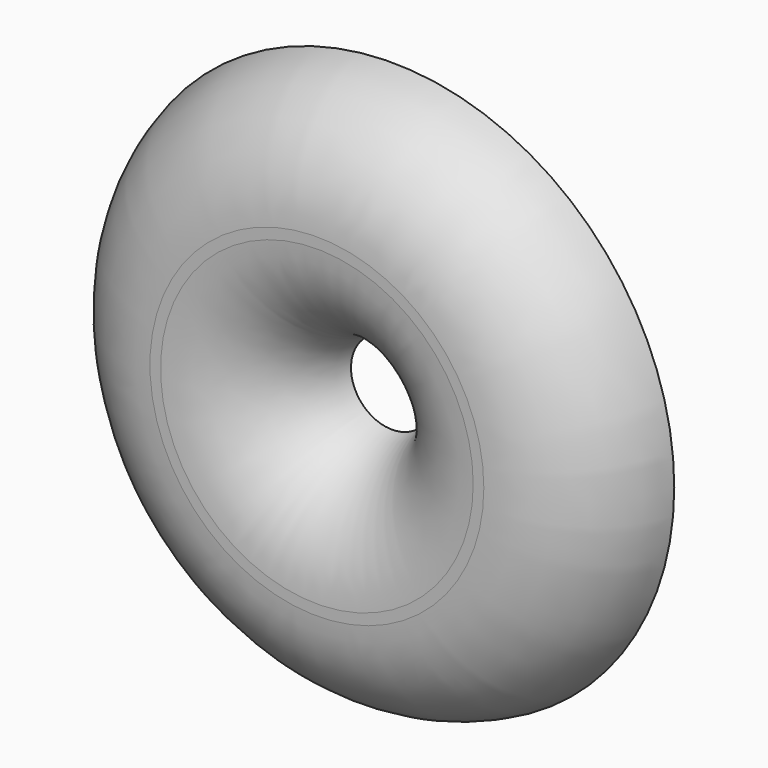
from build123d import *

# Parameters (mm, degrees)
F0_R     = 12
F0_R_2   = 1.75
F1_DEPTH = 4


# Not quite as in the source:
# - a fillet or chamfer that OpenCascade refuses, or shapes differently, is made with other operations: its cross-section is extruded or revolved along the edge and cut away or added


with BuildPart() as f1:
    # F0 (on Front) → F1 (new body)
    with BuildSketch(Plane.XZ):
        Circle(F0_R)
        Circle(F0_R_2, mode=Mode.SUBTRACT)
    extrude(amount=F1_DEPTH)

    # F2: fillet of radius 5 on 2 edges, made by hand

    # F2_s1 → F2_t2 (revolve, cut)
    with BuildSketch(Plane.XY):
        with BuildLine():
            ThreePointArc((12, 0), (10.2632981746, -2.8729833462), (7.1010205144, -4))
            Line((7.1010205144, -4), (12, -4))
            Line((12, -4), (12, 0))
        make_face()
    revolve(axis=Axis((0, -4, 0), (0, -1, 0)), mode=Mode.SUBTRACT)

    # F2_s3 → F2_t4 (revolve, cut)
    with BuildSketch(Plane.XY):
        with BuildLine():
            ThreePointArc((1.75, 0), (3.4867018254, -2.8729833462), (6.6489794856, -4))
            Line((6.6489794856, -4), (1.75, -4))
            Line((1.75, -4), (1.75, 0))
        make_face()
    revolve(axis=Axis((0, -4, 0), (0, -1, 0)), mode=Mode.SUBTRACT)


solid = f1.part
